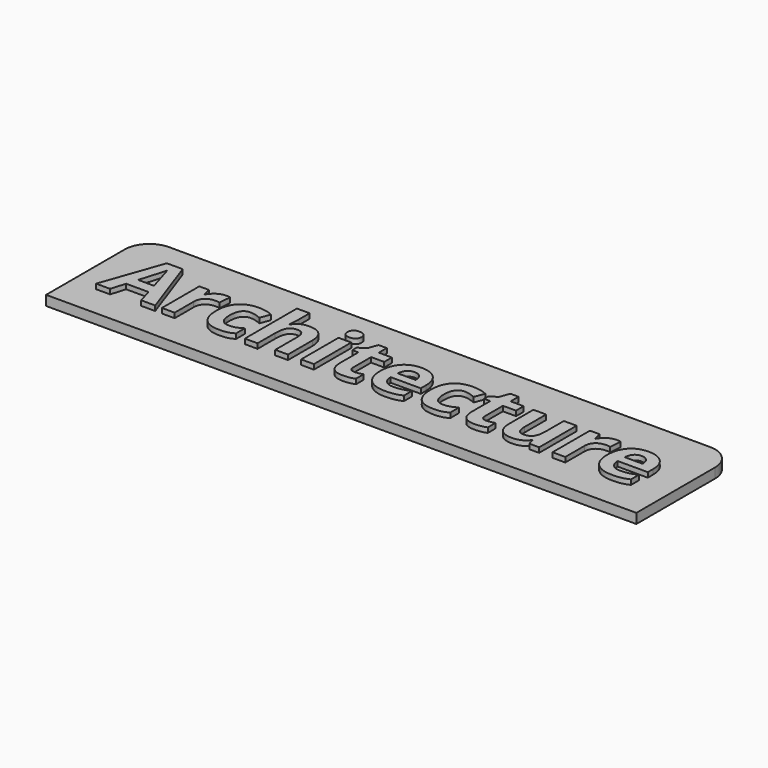
from build123d import *

# Parameters (mm, degrees)
F0_W         = 120
F0_H         = 25
F1_DEPTH     = 2
F2_TEXT_SIZE = 17.4115202928
F3_DEPTH     = 1
F4_R         = 5


# Not quite as in the source:
# - Text() gives the source's letters only with a copy of the font that has no kerning and outlines rounded to 1/6400 em; it was checked with that copy


with BuildPart() as f1:
    # F0 (on Top) → F1 (new body)
    with BuildSketch(Plane.XY):
        Rectangle(F0_W, F0_H)
    extrude(amount=F1_DEPTH)

    # F2 (on face) → F3 (join)
    with BuildSketch(Plane.XY.offset(2)):
        with Locations((-55, -6.0362946108)):
            Text('Architecture', F2_TEXT_SIZE, font='Open Sans', font_style=FontStyle.BOLD, text_align=(TextAlign.LEFT, TextAlign.BOTTOM))
    extrude(amount=F3_DEPTH)

    # F4
    f4_edges = [f1.edges().sort_by_distance(p)[0] for p in [
        (-60, 12.5, 1),
        (60, 12.5, 1),
    ]]
    fillet(f4_edges, radius=F4_R)


solid = f1.part
